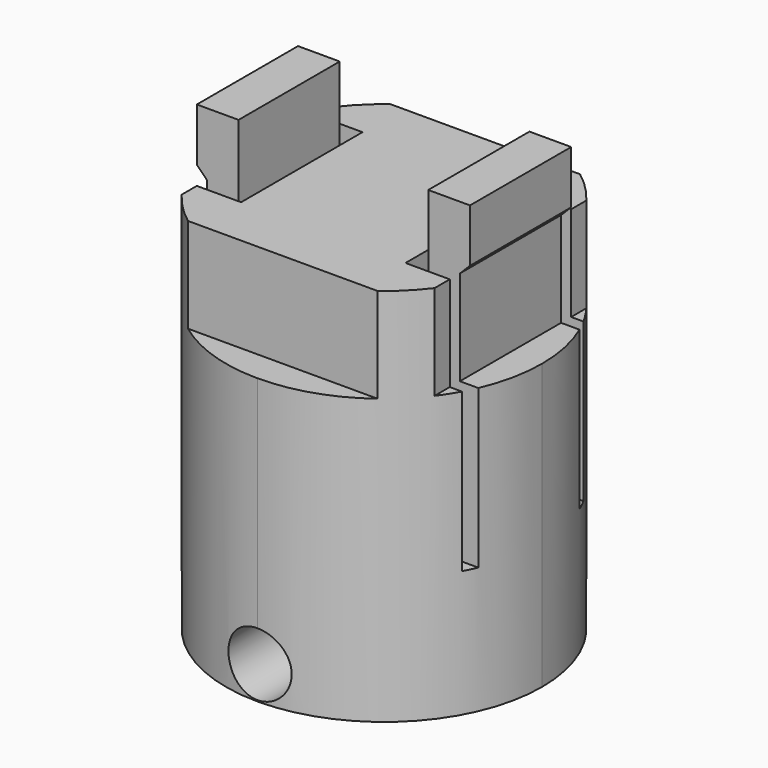
from build123d import *

# Parameters (mm, degrees)
F0_W      = 31.75
F0_H      = 31.75
F0_R      = 4.2545
F1_DEPTH  = 38.1
F2_R      = 1.27
F3_DEPTH  = 76.2
F2_R_2    = 3.175
F4_DEPTH  = 6.35
F6_W      = 31.75
F6_H      = 31.75
F6_W_2    = 25.4
F6_H_2    = 25.4
F7_DEPTH  = 9.525
F8_DEPTH  = 101.6
F9_W      = 3.175
F9_H      = 1.27
F9_W_2    = 1.27
F9_H_2    = 12.7
F10_DEPTH = 25.4
F11_W     = 3.175
F11_H     = 12.7
F11_W_2   = 1.016
F11_W_3   = 4.191
F12_DEPTH = 6.35
F13_SIZE  = 1.01599
F14_W     = 12.7
F14_H     = 12.7
F14_R     = 4.2545
F15_DEPTH = 12.7
F16_SIZE  = 4.1275


# Not quite as in the source:
# - a fillet or chamfer is up to 0.001 mm smaller than in the source, because OpenCascade refuses the exact size


with BuildPart() as f1:
    # F0 (on Top) → F1 (new body)
    with BuildSketch(Plane.XY):
        Rectangle(F0_W, F0_H)
        Circle(F0_R, mode=Mode.SUBTRACT)
    extrude(amount=F1_DEPTH)

    # F2 (on face) → F3 (cut)
    with BuildSketch(Plane.XZ.offset(15.875)):
        with Locations((0, 3.302)):
            Circle(F2_R)
    extrude(amount=-F3_DEPTH, mode=Mode.SUBTRACT)

    # F2 (on face) → F4 (cut)
    with BuildSketch(Plane.XZ.offset(15.875)):
        with Locations((0, 3.302)):
            Circle(F2_R_2)
        with Locations((0, 3.302)):
            Circle(F2_R, mode=Mode.SUBTRACT)
    extrude(amount=-F4_DEPTH, mode=Mode.SUBTRACT)

    # F6 (on face) → F7 (cut)
    with BuildSketch(Plane.XY.offset(38.1)):
        Rectangle(F6_W, F6_H)
        Rectangle(F6_W_2, F6_H_2, mode=Mode.SUBTRACT)
    extrude(amount=-F7_DEPTH, mode=Mode.SUBTRACT)

    # F5 (on face) → F8 (cut)
    with BuildSketch(Plane(origin=(0, 0, 0), x_dir=(1, 0, 0), z_dir=(0, 0, -1))):
        with BuildLine():
            Line((15.875, -15.875), (15.875, 0))
            ThreePointArc((15.875, 0), (11.2253201706, -11.2253201321), (5.44e-08, -15.875))
            Line((5.44e-08, -15.875), (15.875, -15.875))
        make_face()
        with BuildLine():
            Line((-15.875, -15.875), (5.44e-08, -15.875))
            ThreePointArc((5.44e-08, -15.875), (-11.2253201321, -11.2253201706), (-15.875, 0))
            Line((-15.875, 0), (-15.875, -15.875))
        make_face()
        with BuildLine():
            ThreePointArc((-15.875, 0), (-11.2253201513, 11.2253201513), (0, 15.875))
            Line((0, 15.875), (-15.875, 15.875))
            Line((-15.875, 15.875), (-15.875, 0))
        make_face()
        with BuildLine():
            ThreePointArc((0, 15.875), (11.2253201513, 11.2253201513), (15.875, 0))
            Line((15.875, 0), (15.875, 15.875))
            Line((15.875, 15.875), (0, 15.875))
        make_face()
    extrude(amount=-F8_DEPTH, mode=Mode.SUBTRACT)

    # F9 (on face) → F10 (cut)
    with BuildSketch(Plane.XY.offset(38.1)):
        with Locations((-14.2875, 6.985)):
            Rectangle(F9_W, F9_H)
        with Locations((-11.1125, 6.985)):
            Rectangle(F9_W, F9_H)
        with Locations((-8.89, 6.985)):
            Rectangle(F9_W_2, F9_H)
        with Locations((-8.89, 0)):
            Rectangle(F9_W_2, F9_H_2)
        with Locations((-8.89, -6.985)):
            Rectangle(F9_W_2, F9_H)
        with Locations((-11.1125, -6.985)):
            Rectangle(F9_W, F9_H)
        with Locations((-14.2875, -6.985)):
            Rectangle(F9_W, F9_H)
        with Locations((14.2875, 6.985)):
            Rectangle(F9_W, F9_H)
        with Locations((11.1125, 6.985)):
            Rectangle(F9_W, F9_H)
        with Locations((8.89, 6.985)):
            Rectangle(F9_W_2, F9_H)
        with Locations((8.89, 0)):
            Rectangle(F9_W_2, F9_H_2)
        with Locations((8.89, -6.985)):
            Rectangle(F9_W_2, F9_H)
        with Locations((11.1125, -6.985)):
            Rectangle(F9_W, F9_H)
        with Locations((14.2875, -6.985)):
            Rectangle(F9_W, F9_H)
    extrude(amount=-F10_DEPTH, mode=Mode.SUBTRACT)

    # F11 (on face) → F12 (join)
    with BuildSketch(Plane.XY.offset(38.1)):
        with Locations((11.1125, 0)):
            Rectangle(F11_W, F11_H)
        with Locations((13.208, 0)):
            Rectangle(F11_W_2, F11_H)
        with Locations((-11.6205, 0)):
            Rectangle(F11_W_3, F11_H)
    extrude(amount=F12_DEPTH)

    # F13 (size 1.016 in the source; OpenCascade refuses exactly that, so slightly less here)
    f13_edges = [f1.edges().sort_by_distance(p)[0] for p in [
        (13.716, 0, 38.1),
        (-13.716, 0, 38.1),
    ]]
    chamfer(f13_edges, length=F13_SIZE)

    # F14 (on face) → F15 (join)
    with BuildSketch(Plane.XY.offset(38.1)):
        Rectangle(F14_W, F14_H)
        Circle(F14_R, mode=Mode.SUBTRACT)
        Circle(F14_R)
    extrude(amount=-F15_DEPTH)

    # F16
    f16_edges = [f1.edges().sort_by_distance(p)[0] for p in [
        (-4.2545, 0, 25.4),
    ]]
    chamfer(f16_edges, length=F16_SIZE)


solid = f1.part
